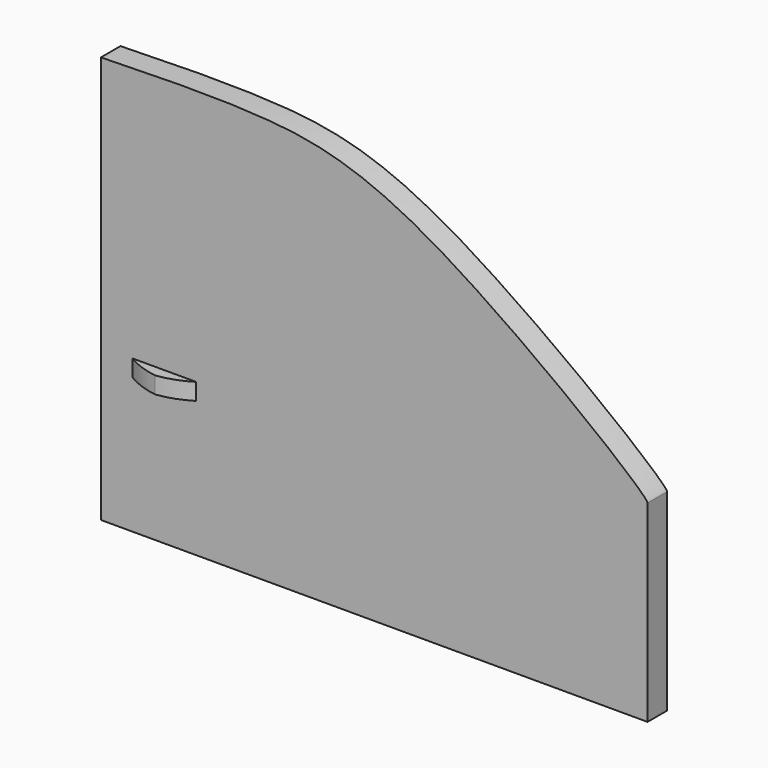
from build123d import *

# Parameters (mm, degrees)
F0_W        = 3.9714416489
F0_H        = 1.0451159906
F1_DEPTH    = 1.524
F2_DEPTH    = 2.286
F3_T1_DEPTH = 14.4253962567


# Not quite as in the source:
# - a fillet or chamfer that OpenCascade refuses, or shapes differently, is made with other operations: its cross-section is extruded or revolved along the edge and cut away or added
# - a feature names something its author has since deleted; it is built from what else it names


with BuildPart() as f1:
    # F0 (on Front) → F1 (new body)
    with BuildSketch(Plane.XZ):
        with BuildLine():
            add(Edge.make_bspline(
                [(-20.49517259, 13.3787927493), (-17.1841776189, 13.4669259304), (-10.2854077584, 13.6505597138), (-0.9687704074, 12.0739679533), (13.6266309982, 0.4298166184), (13.5977584869, 0)],
                knots=[0, 0, 0, 0, 0.2817116399, 0.5869727341, 0.9597554024, 0.9597554024, 0.9597554024, 0.9597554024], degree=3))
            Line((-20.49517259, 13.3787927493), (-20.49517259, 0))
            Line((-20.49517259, 0), (13.4006887674, 0))
            Line((13.4006887674, 0), (13.5977584869, 0))
        make_face()
        with BuildLine():
            add(Edge.make_bspline(
                [(13.5977584869, 0), (13.5946414895, -0.0464018269), (13.4976651285, -0.0232009135), (13.4006887674, 0)],
                knots=[0.9597554024, 0.9597554024, 0.9597554024, 0.9597554024, 1, 1, 1, 1], degree=3))
            Line((13.5977584869, 0), (13.4006887674, 0))
        make_face()
        with BuildLine():
            Line((13.4006887674, 0), (-20.49517259, 0))
            Line((-20.49517259, 0), (-20.49517259, -12.0212072507))
            Line((-20.49517259, -12.0212072507), (13.5977584869, -12.0212072507))
            Line((13.5977584869, -12.0212072507), (13.5977584869, 0))
            add(Edge.make_bspline(
                [(13.5977584869, 0), (13.5946414895, -0.0464018269), (13.4976651285, -0.0232009135), (13.4006887674, 0)],
                knots=[0.9597554024, 0.9597554024, 0.9597554024, 0.9597554024, 1, 1, 1, 1], degree=3))
        make_face()
        with Locations((-16.535716597, -3.0308364658)):
            Rectangle(F0_W, F0_H, mode=Mode.SUBTRACT)
    extrude(amount=F1_DEPTH)

    # F0 (on Front) → F2 (join)
    with BuildSketch(Plane.XZ):
        with Locations((-16.535716597, -3.0308364658)):
            Rectangle(F0_W, F0_H)
    extrude(amount=F2_DEPTH)

    # F3: fillet of radius 5.08 on 2 edges, made by hand

    # F3_s2 → F3_t1 (cut)
    with BuildSketch(Plane.XY.offset(-10.2435345941)):
        with BuildLine():
            ThreePointArc((-18.5214374214, -1.524), (-17.2365966643, -2.0917875517), (-15.8453813682, -2.286))
            Line((-15.8453813682, -2.286), (-18.5214374214, -2.286))
            Line((-18.5214374214, -2.286), (-18.5214374214, -1.524))
        make_face()
        with BuildLine():
            ThreePointArc((-14.5499957725, -1.524), (-15.8348365297, -2.0917875517), (-17.2260518258, -2.286))
            Line((-17.2260518258, -2.286), (-14.5499957725, -2.286))
            Line((-14.5499957725, -2.286), (-14.5499957725, -1.524))
        make_face()
    extrude(amount=F3_T1_DEPTH, mode=Mode.SUBTRACT)


solid = f1.part
